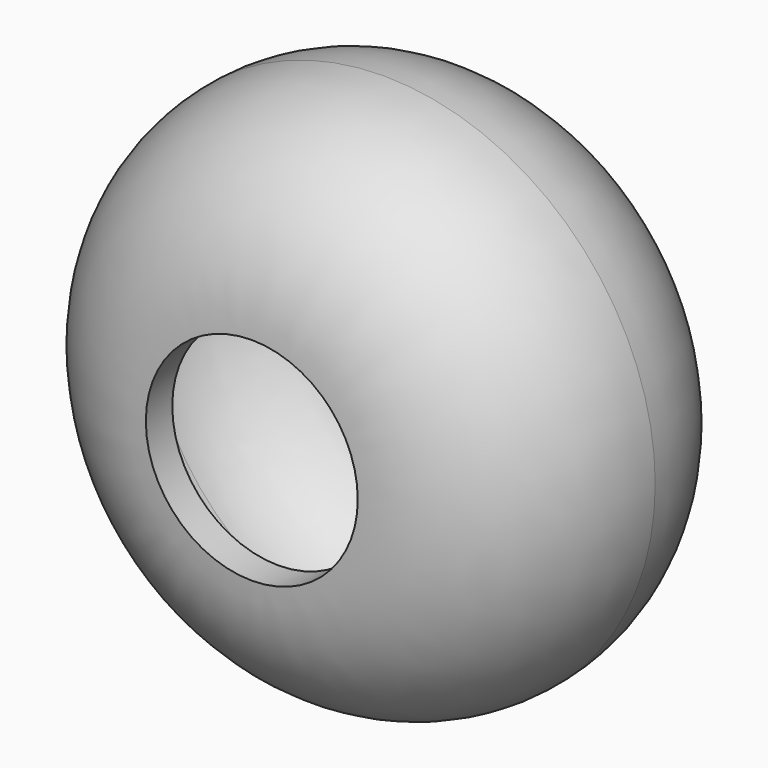
from build123d import *

# Parameters (mm, degrees)
F0_R     = 20.8431321475
F1_DEPTH = 25.4
F2_R     = 12.69999
F3_T     = -2.54
F4_R     = 8.1431421475
F5_DEPTH = 25.4


# Not quite as in the source:
# - a fillet or chamfer is up to 0.001 mm smaller than in the source, because OpenCascade refuses the exact size


with BuildPart() as f1:
    # F0 (on Front) → F1 (new body)
    with BuildSketch(Plane.XZ):
        with Locations((-29.677150771, 16.4469685405)):
            Circle(F0_R)
    extrude(amount=F1_DEPTH)

    # F2 (radius 12.7 in the source; OpenCascade refuses exactly that, so slightly less here)
    f2_edges = [f1.edges().sort_by_distance(p)[0] for p in [
        (-50.520283, -25.4, 16.446969),
        (-8.834019, -12.7, 16.446969),
        (-50.520283, 0, 16.446969),
    ]]
    fillet(f2_edges, radius=F2_R)

    # F3: a shell. OpenCascade refuses it in one call, so the cavity is built on its own and cut out:
    # the body offset inwards by the wall thickness, plus a prism from it out through each open face.
    f3_core = offset(f1.part, amount=F3_T, mode=Mode.PRIVATE)
    f3_exits = [f3_core.faces().sort_by_distance(p)[0] for p in [
        (-29.677151, -2.54, 16.446969),
    ]]
    add(f3_core, mode=Mode.SUBTRACT)
    extrude(f3_exits, amount=-F3_T, mode=Mode.SUBTRACT)

    # F4 (on face) → F5 (cut)
    with BuildSketch(Plane(origin=(0, -22.86, 0), x_dir=(-1, 0, 0), z_dir=(0, 1, 0))):
        with Locations((29.677150771, 16.4469685405)):
            Circle(F4_R)
    extrude(amount=-F5_DEPTH, mode=Mode.SUBTRACT)


solid = f1.part
